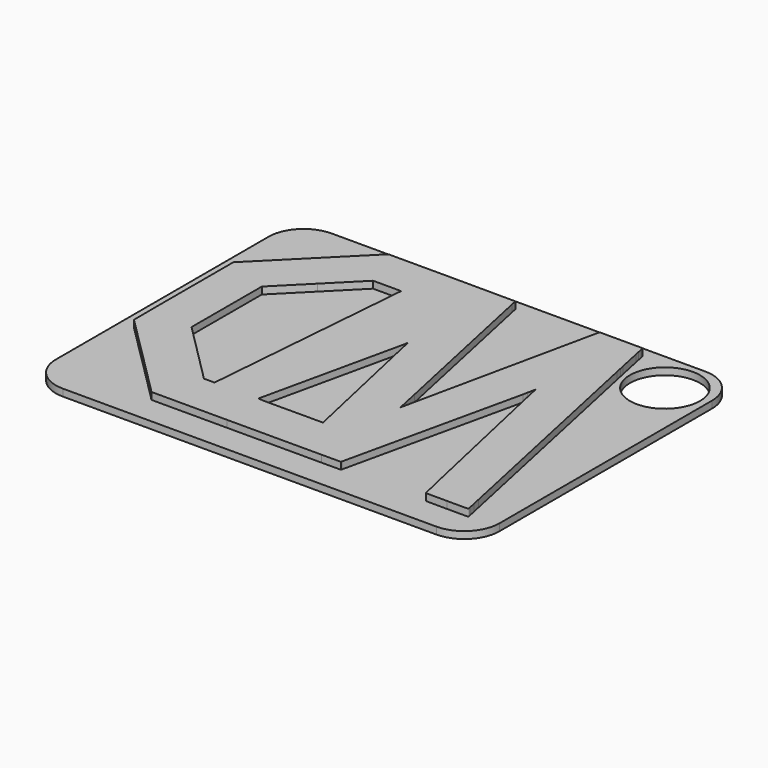
from build123d import *

# Parameters (mm, degrees)
F1_DEPTH = 2
F3_DEPTH = 2
F4_R     = 10
F5_DEPTH = 2


# Not quite as in the source:
# - ends of sketch curves that miss each other by under 0.0002 mm in the source are joined


with BuildPart() as f1:
    # F0 (on Top) → F1 (new body)
    with BuildSketch(Plane.XY):
        with BuildLine():
            Line((-57.600874, 39.53975), (-57.610532, 21.78092))
            add(Edge.make_bspline(
                [(-57.556676, 4.021483), (-57.591601, 4.021748), (-57.615837, 12.013561), (-57.610532, 21.78092)],
                knots=[0, 0, 0, 0, 1, 1, 1, 1], degree=3))
            add(Edge.make_bspline(
                [(-40.075238, -13.389783), (-52.206941, -1.240682), (-57.489675, 4.020846), (-57.556676, 4.021483)],
                knots=[0, 0, 0, 0, 1, 1, 1, 1], degree=3))
            Line((-40.075238, -13.389783), (-32.732625, -20.74289))
            Line((-32.732625, -20.74289), (-11.246228, -20.737043))
            add(Edge.make_bspline(
                [(15.761272, -20.715876), (12.72466, -20.724263), (0.571289, -20.733815), (-11.246228, -20.737043)],
                knots=[0, 0, 0, 0, 1, 1, 1, 1], degree=3))
            Line((15.761272, -20.715876), (21.282367, -20.700583))
            Line((21.282367, -20.700583), (21.365348, -20.383083))
            Line((21.365348, -20.383083), (32.636497, 30.01475))
            add(Edge.make_bspline(
                [(32.894223, 31.327084), (32.850424, 31.047684), (32.734449, 30.457134), (32.636497, 30.01475)],
                knots=[0, 0, 0, 0, 1, 1, 1, 1], degree=3))
            add(Edge.make_bspline(
                [(33.065223, 32.17375), (33.014973, 31.987484), (32.938019, 31.606484), (32.894223, 31.327084)],
                knots=[0, 0, 0, 0, 1, 1, 1, 1], degree=3))
            add(Edge.make_bspline(
                [(33.244505, 33.048222), (33.196152, 32.753529), (33.115473, 32.360017), (33.065223, 32.17375)],
                knots=[0, 0, 0, 0, 1, 1, 1, 1], degree=3))
            add(Edge.make_bspline(
                [(33.393587, 33.513889), (33.35994, 33.552468), (33.292857, 33.342918), (33.244505, 33.048222)],
                knots=[0, 0, 0, 0, 1, 1, 1, 1], degree=3))
            add(Edge.make_bspline(
                [(33.592469, 32.68175), (33.516716, 33.10085), (33.427223, 33.475313), (33.393587, 33.513889)],
                knots=[0, 0, 0, 0, 1, 1, 1, 1], degree=3))
            add(Edge.make_bspline(
                [(33.853308, 31.369417), (33.785593, 31.6721), (33.668211, 32.26265), (33.592469, 32.68175)],
                knots=[0, 0, 0, 0, 1, 1, 1, 1], degree=3))
            add(Edge.make_bspline(
                [(34.24613, 29.591417), (34.097794, 30.266634), (33.921026, 31.066734), (33.853308, 31.369417)],
                knots=[0, 0, 0, 0, 1, 1, 1, 1], degree=3))
            add(Edge.make_bspline(
                [(34.642132, 27.813417), (34.572663, 28.1161), (34.394466, 28.9162), (34.24613, 29.591417)],
                knots=[0, 0, 0, 0, 1, 1, 1, 1], degree=3))
            Line((34.642132, 27.813417), (43.963829, -14.138916))
            add(Edge.make_bspline(
                [(44.826481, -17.86425), (44.411157, -15.981406), (44.235923, -15.22469), (43.963829, -14.138916)],
                knots=[0, 0, 0, 0, 1, 1, 1, 1], degree=3))
            add(Edge.make_bspline(
                [(45.416177, -20.446583), (45.347208, -20.200915), (45.191818, -19.52048), (44.826481, -17.86425)],
                knots=[0, 0, 0, 0, 1, 1, 1, 1], degree=3))
            Line((45.416177, -20.446583), (45.475594, -20.65825))
            Line((45.475594, -20.65825), (51.543384, -20.679972))
            add(Edge.make_bspline(
                [(57.611164, -20.530527), (57.611164, -20.700927), (57.583613, -20.701604), (51.543384, -20.679972)],
                knots=[0, 0, 0, 0, 1, 1, 1, 1], degree=3))
            add(Edge.make_bspline(
                [(57.486095, -19.873802), (57.554887, -20.140857), (57.611164, -20.436386), (57.611164, -20.530527)],
                knots=[0, 0, 0, 0, 1, 1, 1, 1], degree=3))
            add(Edge.make_bspline(
                [(57.057166, -17.90658), (57.224288, -18.721497), (57.417304, -19.606745), (57.486095, -19.873802)],
                knots=[0, 0, 0, 0, 1, 1, 1, 1], degree=3))
            add(Edge.make_bspline(
                [(56.632883, -15.87458), (56.699119, -16.177264), (56.890042, -17.091664), (57.057166, -17.90658)],
                knots=[0, 0, 0, 0, 1, 1, 1, 1], degree=3))
            Line((56.632883, -15.87458), (42.202773, 51.604753))
            add(Edge.make_bspline(
                [(41.814745, 53.403919), (41.881251, 53.089594), (42.055857, 52.27997), (42.202773, 51.604753)],
                knots=[0, 0, 0, 0, 1, 1, 1, 1], degree=3))
            add(Edge.make_bspline(
                [(41.571733, 54.546919), (41.638893, 54.232594), (41.748247, 53.718244), (41.814745, 53.403919)],
                knots=[0, 0, 0, 0, 1, 1, 1, 1], degree=3))
            add(Edge.make_bspline(
                [(40.19839, 61.002752), (40.407617, 60.004619), (40.846698, 57.940575), (41.571733, 54.546919)],
                knots=[0, 0, 0, 0, 1, 1, 1, 1], degree=3))
            add(Edge.make_bspline(
                [(39.946549, 62.188085), (40.011853, 61.885402), (40.12518, 61.352002), (40.19839, 61.002752)],
                knots=[0, 0, 0, 0, 1, 1, 1, 1], degree=3))
            add(Edge.make_bspline(
                [(39.691567, 63.436919), (39.766505, 63.052744), (39.881255, 62.490769), (39.946549, 62.188085)],
                knots=[0, 0, 0, 0, 1, 1, 1, 1], degree=3))
            Line((39.691567, 63.436919), (39.55532, 64.135419))
            Line((39.55532, 64.135419), (33.389412, 64.135419))
            Line((33.389412, 64.135419), (27.223504, 64.135419))
            Line((27.223504, 64.135419), (27.169883, 63.817919))
            add(Edge.make_bspline(
                [(27.003116, 62.992419), (27.065346, 63.271819), (27.140385, 63.643294), (27.169883, 63.817919)],
                knots=[0, 0, 0, 0, 1, 1, 1, 1], degree=3))
            Line((27.003116, 62.992419), (15.335584, 8.551753))
            Line((15.335584, 8.551753), (15.226041, 8.043753))
            Line((15.226041, 8.043753), (15.121547, 8.594086))
            add(Edge.make_bspline(
                [(14.902964, 9.65242), (14.96571, 9.37302), (15.064074, 8.89677), (15.121547, 8.594086)],
                knots=[0, 0, 0, 0, 1, 1, 1, 1], degree=3))
            add(Edge.make_bspline(
                [(14.65394, 10.79542), (14.728159, 10.44617), (14.840215, 9.93182), (14.902964, 9.65242)],
                knots=[0, 0, 0, 0, 1, 1, 1, 1], degree=3))
            add(Edge.make_bspline(
                [(13.790663, 14.85942), (13.90813, 14.305525), (14.109002, 13.359899), (14.65394, 10.79542)],
                knots=[0, 0, 0, 0, 1, 1, 1, 1], degree=3))
            Line((13.790663, 14.85942), (3.603226, 62.399752))
            add(Edge.make_bspline(
                [(3.255508, 64.071919), (3.255677, 64.036994), (3.41217, 63.284519), (3.603226, 62.399752)],
                knots=[0, 0, 0, 0, 1, 1, 1, 1], degree=3))
            add(Edge.make_bspline(
                [(-14.888194, 64.135419), (-4.909346, 64.135419), (3.25532, 64.106844), (3.255508, 64.071919)],
                knots=[0, 0, 0, 0, 1, 1, 1, 1], degree=3))
            Line((-14.888194, 64.135419), (-33.031551, 64.135419))
            Line((-33.031551, 64.135419), (-35.398694, 61.752788))
            add(Edge.make_bspline(
                [(-47.683354, 49.454953), (-42.228717, 54.908316), (-36.700618, 60.442341), (-35.398694, 61.752788)],
                knots=[0, 0, 0, 0, 1, 1, 1, 1], degree=3))
            Line((-47.683354, 49.454953), (-57.600874, 39.53975))
        make_face()
        with BuildLine():
            Line((6.375168, -8.424191), (0.221996, -8.424191))
            add(Edge.make_bspline(
                [(-7.243511, -8.453309), (-6.521727, -8.43746), (-3.162249, -8.424353), (0.221996, -8.424191)],
                knots=[0, 0, 0, 0, 1, 1, 1, 1], degree=3))
            add(Edge.make_bspline(
                [(-12.154177, -8.326219), (-12.154177, -8.432404), (-9.462714, -8.502061), (-7.243511, -8.453309)],
                knots=[0, 0, 0, 0, 1, 1, 1, 1], degree=3))
            add(Edge.make_bspline(
                [(-12.074445, -7.925738), (-12.118297, -8.094121), (-12.154177, -8.274339), (-12.154177, -8.326219)],
                knots=[0, 0, 0, 0, 1, 1, 1, 1], degree=3))
            Line((-12.074445, -7.925738), (-3.125565, 32.382041))
            add(Edge.make_bspline(
                [(-3.010177, 33.024095), (-3.010177, 32.925223), (-3.062102, 32.636298), (-3.125565, 32.382041)],
                knots=[0, 0, 0, 0, 1, 1, 1, 1], degree=3))
            add(Edge.make_bspline(
                [(-2.787964, 32.835209), (-2.881087, 33.302508), (-3.010177, 33.412077), (-3.010177, 33.024095)],
                knots=[0, 0, 0, 0, 1, 1, 1, 1], degree=3))
            add(Edge.make_bspline(
                [(-2.284888, 30.480139), (-2.479074, 31.355119), (-2.685944, 32.323547), (-2.787964, 32.835209)],
                knots=[0, 0, 0, 0, 1, 1, 1, 1], degree=3))
            Line((-2.284888, 30.480139), (6.006286, -6.900191))
            add(Edge.make_bspline(
                [(6.260018, -7.979691), (6.196685, -7.735216), (6.082504, -7.249441), (6.006286, -6.900191)],
                knots=[0, 0, 0, 0, 1, 1, 1, 1], degree=3))
            Line((6.260018, -7.979691), (6.375168, -8.424191))
        make_face(mode=Mode.SUBTRACT)
        Polygon((-27.716271, 52.028087), (-19.709447, 52.028087), (-24.603371, -8.423914), (-26.117335, -8.423914), (-27.631297, -8.423914), (-36.487388, 0.43695), (-45.343476, 9.297817), (-45.318269, 34.333354), (-36.51727, 43.180719), align=None, mode=Mode.SUBTRACT)
    extrude(amount=F1_DEPTH)


with BuildPart() as f3:
    # F2 (on face) → F3 (new body)
    with BuildSketch(Plane(origin=(0, 0, 0), x_dir=(1, 0, 0), z_dir=(0, 0, -1))):
        with BuildLine():
            ThreePointArc((-61.5682080388, -57.0710578561), (-58.6392758507, -64.1421256679), (-51.5682080388, -67.0710578561))
            Line((-51.5682080388, -67.0710578561), (55.0194212794, -67.0710578561))
            ThreePointArc((55.0194212794, -67.0710578561), (62.0904890913, -64.1421256679), (65.0194212794, -57.0710578561))
            Line((65.0194212794, -57.0710578561), (65.0194212794, 18.8257021457))
            ThreePointArc((65.0194212794, 18.8257021457), (62.0904890913, 25.8967699576), (55.0194212794, 28.8257021457))
            Line((55.0194212794, 28.8257021457), (-51.5682080388, 28.8257021457))
            ThreePointArc((-51.5682080388, 28.8257021457), (-58.6392758507, 25.8967699576), (-61.5682080388, 18.8257021457))
            Line((-61.5682080388, 18.8257021457), (-61.5682080388, -57.0710578561))
        make_face()
    extrude(amount=F3_DEPTH)

    # F4 (on face) → F5 (cut)
    with BuildSketch(Plane.XY):
        with Locations((53.0357174575, 55.2100874484)):
            Circle(F4_R)
    extrude(amount=-F5_DEPTH, mode=Mode.SUBTRACT)


solid = Compound([f1.part, f3.part])
